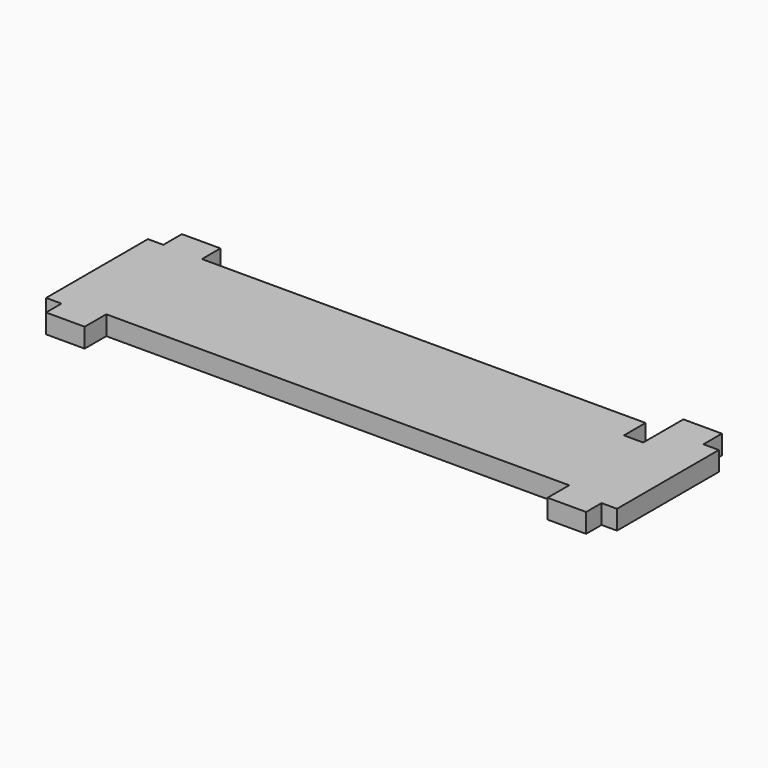
from build123d import *

# Parameters (mm, degrees)
F0_W      = 140
F0_H      = 30
F1_DEPTH  = 5
F2_W      = 10
F2_H      = 5
F3_DEPTH  = 5
F2_H_2    = 9
F5_W      = 5
F5_H      = 8
F6_DEPTH  = 25
F7_W      = 120
F7_H      = 2
F8_DEPTH  = 5
F9_W      = 115
F9_H      = 1
F10_DEPTH = 25
F11_W     = 4
F11_H     = 33
F12_DEPTH = 5


# Not quite as in the source:
# - a feature names something its author has since deleted; it is built from what else it names


with BuildPart() as f1:
    # F0 (on Top) → F1 (new body)
    with BuildSketch(Plane.XY):
        Rectangle(F0_W, F0_H)
    extrude(amount=F1_DEPTH)


with BuildPart() as f3:
    # F2 (on face) → F3 (new body)
    with BuildSketch(Plane.XY.offset(5)):
        with Locations((65, 17.5)):
            Rectangle(F2_W, F2_H)
    extrude(amount=-F3_DEPTH)


with BuildPart() as f3b:
    # F2 (on face) → F3, piece 2 (new body)
    with BuildSketch(Plane.XY.offset(5)):
        with Locations((-65, 17.5)):
            Rectangle(F2_W, F2_H)
    extrude(amount=-F3_DEPTH)


with BuildPart() as f3c:
    # F2 (on face) → F3, piece 3 (new body)
    with BuildSketch(Plane.XY.offset(5)):
        with Locations((-65, -19.5)):
            Rectangle(F2_W, F2_H_2)
    extrude(amount=-F3_DEPTH)


with BuildPart() as f3d:
    # F2 (on face) → F3, piece 4 (new body)
    with BuildSketch(Plane.XY.offset(5)):
        with Locations((65, -19.5)):
            Rectangle(F2_W, F2_H_2)
    extrude(amount=-F3_DEPTH)


with BuildPart() as f3b_1:
    add(f3b.part)

    # F4: union F3, F3c, F3d, F1
    add(f3.part)
    add(f3c.part)
    add(f3d.part)
    add(f1.part)

    # F5 (on face) → F6 (cut)
    with BuildSketch(Plane.XY.offset(5)):
        with Locations((57.5, 11)):
            Rectangle(F5_W, F5_H)
    extrude(amount=-F6_DEPTH, mode=Mode.SUBTRACT)

    # F7 (on face) → F8 (join)
    with BuildSketch(Plane.XY.offset(5)):
        with Locations((0, -16)):
            Rectangle(F7_W, F7_H)
    extrude(amount=-F8_DEPTH)

    # F9 (on face) → F10 (cut)
    with BuildSketch(Plane.XY.offset(5)):
        with Locations((-2.5, 14.5)):
            Rectangle(F9_W, F9_H)
    extrude(amount=-F10_DEPTH, mode=Mode.SUBTRACT)

    # F11 (on Top) → F12 (join)
    with BuildSketch(Plane.XY):
        with Locations((-72, -2.5)):
            Rectangle(F11_W, F11_H)
        with Locations((72, -2.5)):
            Rectangle(F11_W, F11_H)
    extrude(amount=F12_DEPTH)


solid = f3b_1.part
